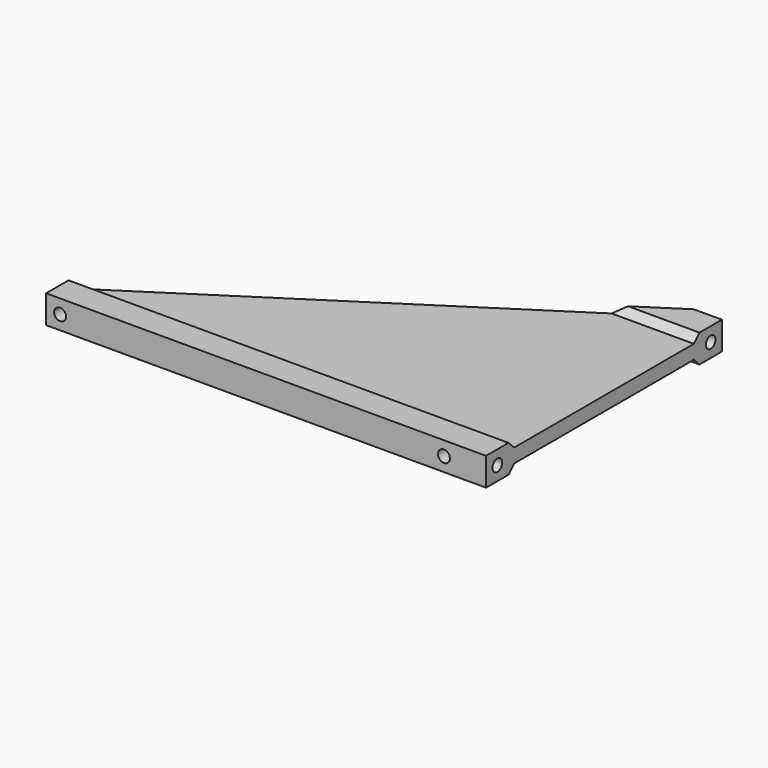
from build123d import *

# Parameters (mm, degrees)
F1_DEPTH = 6.35
F2_R     = 1.35255
F3_DEPTH = 4.7625
F4_R     = 1.35255
F5_DEPTH = 4.7625
F6_W     = 53.975
F6_H     = 1.5875
F7_DEPTH = 99.4996370206
F8_SIZE  = 1.58749


# Not quite as in the source:
# - a fillet or chamfer is up to 0.001 mm smaller than in the source, because OpenCascade refuses the exact size


with BuildPart() as f1:
    # F0 (on Top) → F1 (new body)
    with BuildSketch(Plane.XY):
        Polygon((0, -66.675), (0, 0), (-6.35, 0), (-99.4986370206, -60.325), (-99.4986370206, -66.675), align=None)
    extrude(amount=F1_DEPTH)

    # F2 (on face) → F3 (cut)
    with BuildSketch(Plane.YZ):
        with Locations((-63.5, 3.175)):
            Circle(F2_R)
        with Locations((-3.175, 3.175)):
            Circle(F2_R)
    extrude(amount=-F3_DEPTH, mode=Mode.SUBTRACT)

    # F4 (on face) → F5 (cut)
    with BuildSketch(Plane.XZ.offset(66.675)):
        with Locations((-96.3236370206, 3.175)):
            Circle(F4_R)
        with Locations((-9.525, 3.175)):
            Circle(F4_R)
    extrude(amount=-F5_DEPTH, mode=Mode.SUBTRACT)

    # F6 (on face) → F7 (cut, through all)
    with BuildSketch(Plane.YZ):
        with Locations((-33.3375, 5.55625)):
            Rectangle(F6_W, F6_H)
        with Locations((-33.3375, 0.79375)):
            Rectangle(F6_W, F6_H)
    extrude(amount=-F7_DEPTH, mode=Mode.SUBTRACT)

    # F8 (size 1.5875 in the source; OpenCascade refuses exactly that, so slightly less here)
    f8_edges = [f1.edges().sort_by_distance(p)[0] for p in [
        (-49.749319, -60.325, 4.7625),
        (-49.749319, -60.325, 1.5875),
        (-8.07756, -6.35, 4.7625),
        (-8.07756, -6.35, 1.5875),
    ]]
    chamfer(f8_edges, length=F8_SIZE)


solid = f1.part
